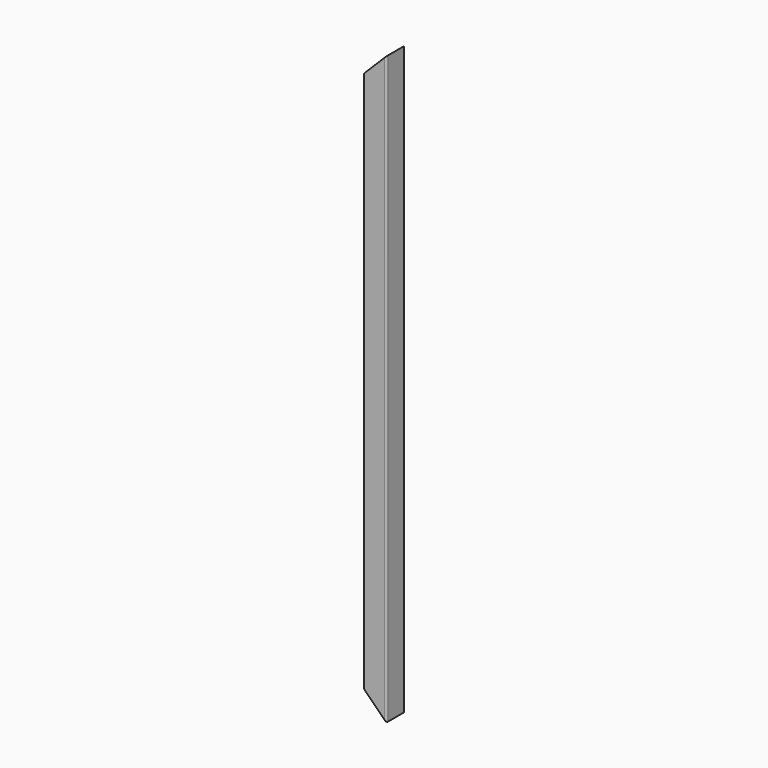
from build123d import *

# Parameters (mm, degrees)
F1_DEPTH      = 500
F3_DEPTH      = 20.001
F3_DEPTH_BACK = 20.001


# Not quite as in the source:
# - a pattern or mirror of a feature is missing from the dataset's text; its kind, count and spacing are read off the source's solid


with BuildPart() as f1:
    # F0 (on Top) → F1 (new body, symmetric)
    with BuildSketch(Plane.XY):
        with BuildLine():
            Line((17, 20), (-17, 20))
            ThreePointArc((-17, 20), (-19.1213203436, 19.1213203436), (-20, 17))
            Line((-20, 17), (-20, -17))
            ThreePointArc((-20, -17), (-19.1213203436, -19.1213203436), (-17, -20))
            Line((-17, -20), (17, -20))
            ThreePointArc((17, -20), (19.1213203436, -19.1213203436), (20, -17))
            Line((20, -17), (20, 17))
            ThreePointArc((20, 17), (19.1213203436, 19.1213203436), (17, 20))
        make_face()
        with BuildLine():
            ThreePointArc((-18, 17), (-17.7071067812, 17.7071067812), (-17, 18))
            Line((-17, 18), (17, 18))
            ThreePointArc((17, 18), (17.7071067812, 17.7071067812), (18, 17))
            Line((18, 17), (18, -17))
            ThreePointArc((18, -17), (17.7071067812, -17.7071067812), (17, -18))
            Line((17, -18), (-17, -18))
            ThreePointArc((-17, -18), (-17.7071067812, -17.7071067812), (-18, -17))
            Line((-18, -17), (-18, 17))
        make_face(mode=Mode.SUBTRACT)
    extrude(amount=F1_DEPTH, both=True)

    # F2 (on Front) → F3 (cut, two sides)
    with BuildSketch(Plane.XZ) as f3_sk:
        Polygon((20, 500), (-20, 500), (-20, 460), align=None)
    f3 = extrude(amount=-F3_DEPTH, mode=Mode.SUBTRACT) + extrude(f3_sk.sketch, amount=F3_DEPTH_BACK, mode=Mode.SUBTRACT)

    # F3_copies: F3 across plane
    add(f3.mirror(Plane(origin=(0, 0, 0), x_dir=(-1, 0, 0), z_dir=(0, 0, -1))), mode=Mode.SUBTRACT)


solid = f1.part
